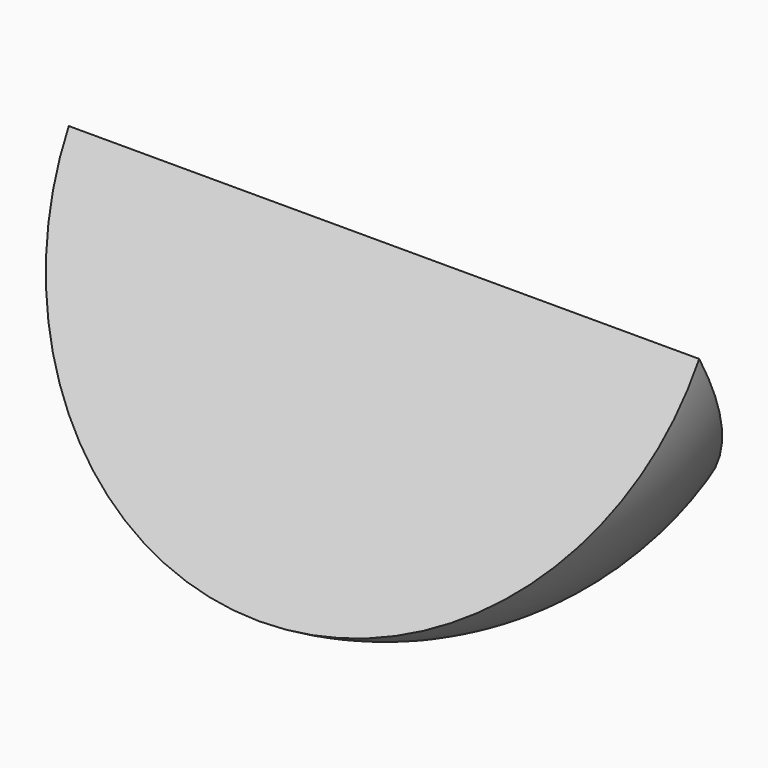
from build123d import *

# Parameters (mm, degrees)
F1_ANGLE_BACK = 30
F1_ANGLE      = 60


with BuildPart() as f1:
    # F0 (on Front) → F1 (revolve)
    with BuildSketch(Plane.XZ, mode=Mode.PRIVATE) as f1_sk:
        with BuildLine():
            Line((39.0365384519, 0), (-41.7184382677, 0))
            ThreePointArc((-41.7184382677, 0), (-1.3409499079, -39.9536792116), (39.0365384519, 0))
        make_face()
    revolve(f1_sk.sketch.rotate(Axis((-1.3409499079, 0, 0), (1, 0, 0)), -F1_ANGLE_BACK), axis=Axis((-1.3409499079, 0, 0), (1, 0, 0)), revolution_arc=F1_ANGLE)


solid = f1.part
